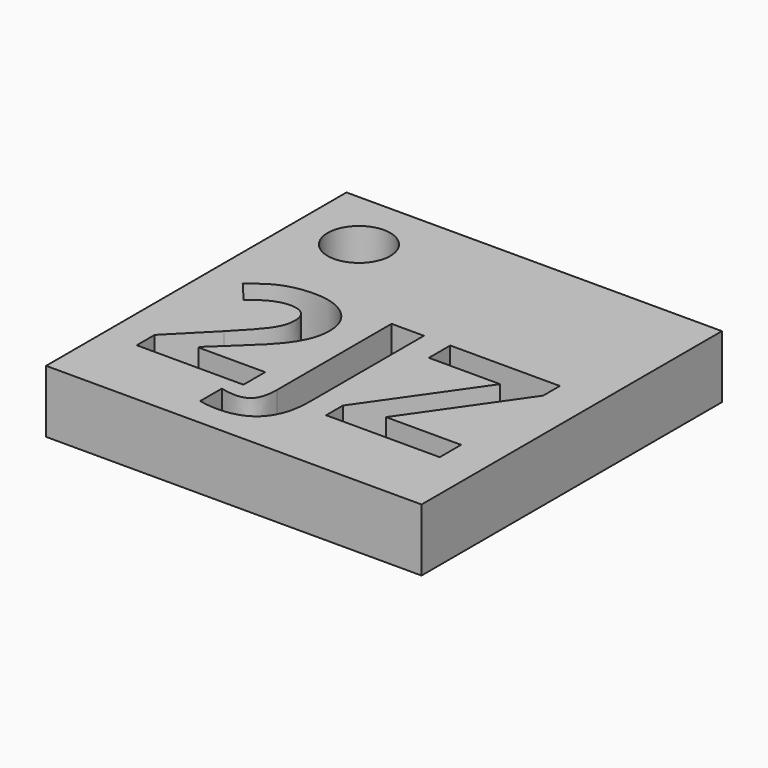
from build123d import *

# Parameters (mm, degrees)
F0_W         = 30
F0_H         = 30
F0_R         = 2.5
F1_DEPTH     = 5
F2_TEXT_SIZE = 17.0841889117
F3_DEPTH     = 5.001


# Not quite as in the source:
# - Text() gives the source's letters only with a copy of the font that has no kerning and outlines rounded to 1/6400 em; it was checked with that copy


with BuildPart() as f1:
    # F0 (on Top) → F1 (new body)
    with BuildSketch(Plane.XY):
        with Locations((15, -15)):
            Rectangle(F0_W, F0_H)
        with Locations((5, -5)):
            Circle(F0_R, mode=Mode.SUBTRACT)
    extrude(amount=F1_DEPTH)

    # F2 (on face) → F3 (cut, through all)
    with BuildSketch(Plane.XY.offset(5)):
        with Locations((2, -24.3006160164)):
            Text('2JZ', F2_TEXT_SIZE, font='Open Sans', font_style=FontStyle.BOLD, text_align=(TextAlign.LEFT, TextAlign.BOTTOM))
    extrude(amount=-F3_DEPTH, mode=Mode.SUBTRACT)


solid = f1.part
